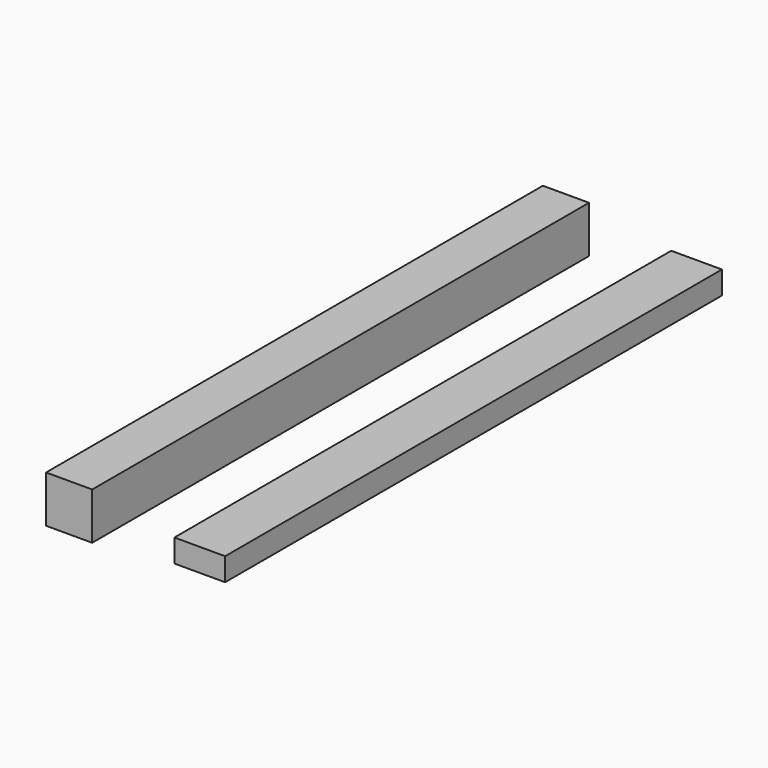
from build123d import *

# Parameters (mm, degrees)
F0_W     = 74.2400288582
F0_H     = 75.5776762962
F1_DEPTH = 1000
F0_W_2   = 81.6530883312
F0_H_2   = 36.9499400258


# Not quite as in the source:
# - a feature of the source that left no trace in its solid (it failed there, or was rolled back) is left out


with BuildPart() as f1:
    # F0 (on Front) → F1 (new body)
    with BuildSketch(Plane.XZ):
        with Locations((-37.1200144291, 37.7888381481)):
            Rectangle(F0_W, F0_H)
    extrude(amount=F1_DEPTH)


with BuildPart() as f1b:
    # F0 (on Front) → F1, piece 2 (new body)
    with BuildSketch(Plane.XZ):
        with Locations((173.2547134161, 32.1330912411)):
            Rectangle(F0_W_2, F0_H_2)
    extrude(amount=F1_DEPTH)


solid = Compound([f1.part, f1b.part])
